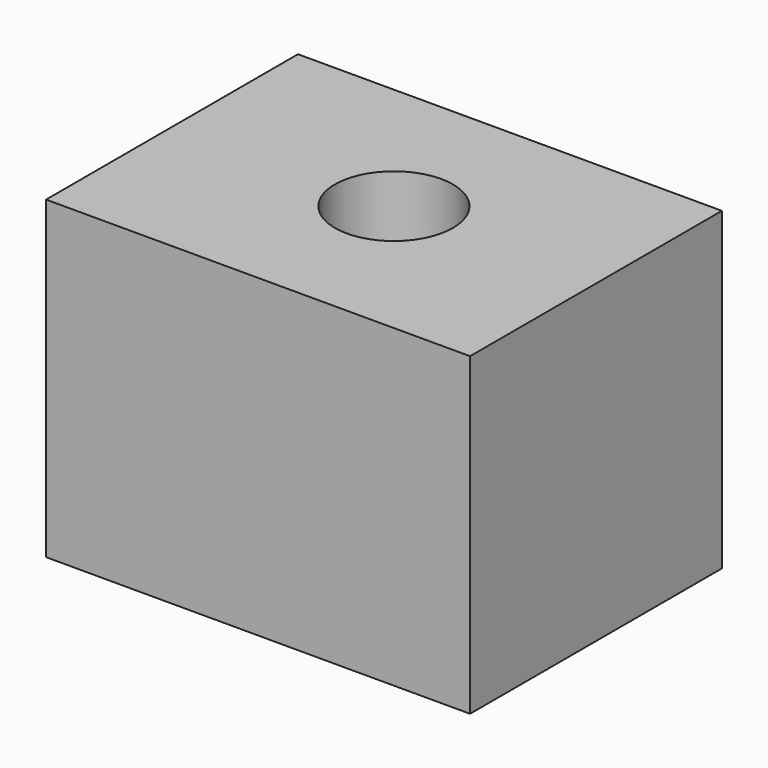
from build123d import *

# Parameters (mm, degrees)
F0_W     = 107.7381369554
F0_H     = 80
F1_DEPTH = 80
F2_R     = 15
F3_DEPTH = 80.001


# Not quite as in the source:
# - a feature names something its author has since deleted; it is built from what else it names


with BuildPart() as f1:
    # F0 (on Top) → F1 (new body)
    with BuildSketch(Plane.XY):
        with Locations((-1.8000006676, -0.9000021964)):
            Rectangle(F0_W, F0_H)
    extrude(amount=F1_DEPTH)

    # F2 (on face) → F3 (cut, through all)
    with BuildSketch(Plane.XY.offset(80)):
        Circle(F2_R)
    extrude(amount=-F3_DEPTH, mode=Mode.SUBTRACT)


solid = f1.part
